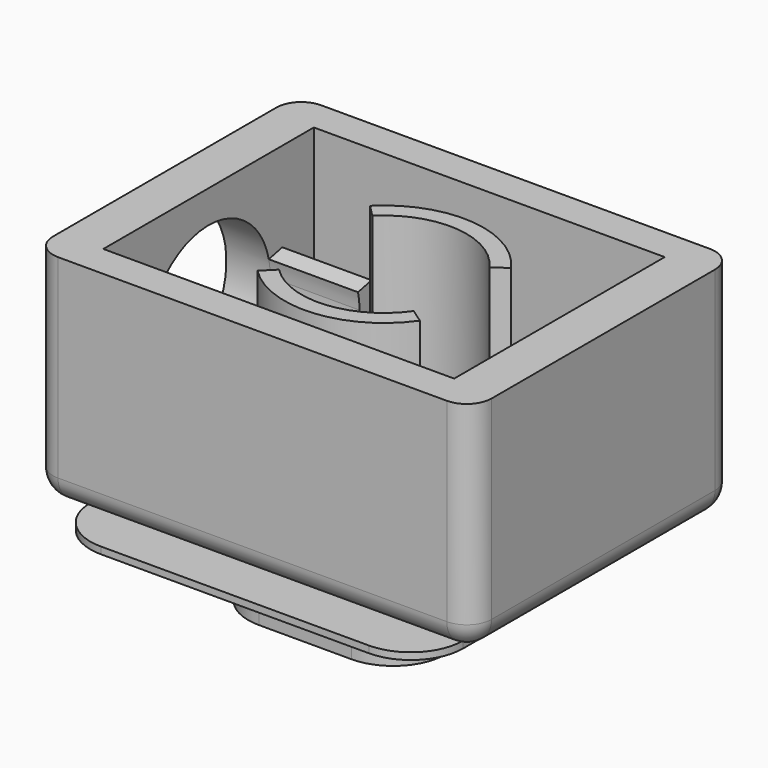
from build123d import *

# Parameters (mm, degrees)
F0_W      = 50.8
F0_H      = 38.1
F1_DEPTH  = 25.4
F2_W      = 40.64
F2_H      = 30.48
F3_DEPTH  = 22.225
F4_R      = 9.5514218063
F5_DEPTH  = 25.4
F6_R      = 8.9260934587
F7_DEPTH  = 25.4
F9_DEPTH  = 10.3378
F11_DEPTH = 21.082
F12_W     = 22.86
F12_H     = 22.86
F12_R     = 10.7189198073
F12_R_2   = 9.5514218063
F13_DEPTH = 9.6266
F14_W     = 22.86
F14_H     = 0.79375
F15_DEPTH = 10.16
F17_DEPTH = 10.16
F18_W     = 10.16
F18_H     = 0.79375
F18_W_2   = 22.86
F19_DEPTH = 10.16
F20_W     = 10.16
F20_H     = 0.79375
F20_W_2   = 22.86
F21_DEPTH = 10.16
F22_R     = 6.0707814239
F23_R     = 2.8820881508


# Not quite as in the source:
# - a length typed as a fraction of an inch, garbled in the dataset ("3 / 203.2 mm" for 3/8 in), is restored
# - a feature names something its author has since deleted; it is built from what else it names


with BuildPart() as f1:
    # F0 (on Top) → F1 (new body)
    with BuildSketch(Plane.XY):
        with Locations((-32.453101594, -1.12241521)):
            Rectangle(F0_W, F0_H)
    extrude(amount=F1_DEPTH)

    # F2 (on face) → F3 (cut)
    with BuildSketch(Plane.XY.offset(25.4)):
        with Locations((-32.453101594, -1.12241521)):
            Rectangle(F2_W, F2_H)
    extrude(amount=-F3_DEPTH, mode=Mode.SUBTRACT)

    # F4 (on face) → F5 (cut)
    with BuildSketch(Plane.XY.offset(3.175)):
        with Locations((-32.453101594, -1.12241521)):
            Circle(F4_R)
    extrude(amount=-F5_DEPTH, mode=Mode.SUBTRACT)

    # F6 (on face) → F7 (cut)
    with BuildSketch(Plane(origin=(-57.853101594, 0, 0), x_dir=(0, -1, 0), z_dir=(-1, 0, 0))):
        with Locations((1.12241521, 12.7)):
            Circle(F6_R)
    extrude(amount=-F7_DEPTH, mode=Mode.SUBTRACT)

    # F8 (on face) → F9 (join)
    with BuildSketch(Plane.YZ.offset(-52.773101594)):
        with BuildLine():
            ThreePointArc((4.2283937472, 3.175), (8.3066529455, 7.1818974988), (9.8026377187, 12.7))
            ThreePointArc((9.8026377187, 12.7), (9.7389872891, 13.8775895924), (9.5487776675, 15.0414576799))
            Line((9.5487776675, 15.0414576799), (7.5962670299, 14.6130406248))
            ThreePointArc((7.5962670299, 14.6130406248), (7.7516739529, 13.6621257514), (7.8036782487, 12.7))
            ThreePointArc((7.8036782487, 12.7), (-3.0308273005, 3.9803034613), (-9.2324659679, 16.4285682425))
            Line((-9.2324659679, 16.4285682425), (-11.0486762552, 17.2635647427))
            ThreePointArc((-11.0486762552, 17.2635647427), (-11.5132347682, 9.3254407095), (-6.4732241672, 3.175))
            Line((-6.4732241672, 3.175), (4.2283937472, 3.175))
        make_face()
    extrude(amount=F9_DEPTH)

    # F10 (on face) → F11 (join)
    with BuildSketch(Plane.XY.offset(3.175)):
        with BuildLine():
            Line((-24.6290348955, 4.3560552717), (-23.0209375751, 5.4820571376))
            ThreePointArc((-23.0209375751, 5.4820571376), (-31.4495427718, 10.3483146168), (-40.5951152599, 7.0195984558))
            Line((-40.5951152599, 7.0195984558), (-39.2069767232, 5.6314599192))
            ThreePointArc((-39.2069767232, 5.6314599192), (-31.6206403322, 8.3926605526), (-24.6290348955, 4.3560552717))
        make_face()
        with BuildLine():
            ThreePointArc((-40.5951152599, -9.2644288759), (-31.4495427718, -12.5931450369), (-23.0209375751, -7.7268875577))
            Line((-23.0209375751, -7.7268875577), (-24.6290348955, -6.6008856918))
            ThreePointArc((-24.6290348955, -6.6008856918), (-31.6206403322, -10.6374909727), (-39.2069767232, -7.8762903393))
            Line((-39.2069767232, -7.8762903393), (-40.5951152599, -9.2644288759))
        make_face()
    extrude(amount=F11_DEPTH)

    # F12 (on face) → F13 (join)
    with BuildSketch(Plane(origin=(0, 0, 0), x_dir=(1, 0, 0), z_dir=(0, 0, -1))):
        with Locations((-32.453101594, 1.12241521)):
            Rectangle(F12_W, F12_H)
        with Locations((-32.453101594, 1.12241521)):
            Circle(F12_R, mode=Mode.SUBTRACT)
        with Locations((-32.453101594, 1.12241521)):
            Circle(F12_R)
        with Locations((-32.453101594, 1.12241521)):
            Circle(F12_R_2, mode=Mode.SUBTRACT)
    extrude(amount=F13_DEPTH)

    # F14 (on face) → F15 (join)
    with BuildSketch(Plane(origin=(0, 10.30758479, 0), x_dir=(-1, 0, 0), z_dir=(0, 1, 0))):
        with Locations((32.453101594, -1.190625)):
            Rectangle(F14_W, F14_H)
    extrude(amount=F15_DEPTH)

    # F16 (on face) → F17 (join)
    with BuildSketch(Plane.YZ.offset(-21.023101594)):
        Polygon((-12.55241521, -0.79375), (-12.55241521, -1.5875), (10.30758479, -1.5875), (20.46758479, -1.5875), (20.46758479, -0.79375), (10.30758479, -0.79375), align=None)
    extrude(amount=F17_DEPTH)

    # F18 (on face) → F19 (join)
    with BuildSketch(Plane.XZ.offset(12.55241521)):
        with Locations((-15.943101594, -1.190625)):
            Rectangle(F18_W, F18_H)
        with Locations((-32.453101594, -1.190625)):
            Rectangle(F18_W_2, F18_H)
    extrude(amount=F19_DEPTH)

    # F20 (on face) → F21 (join)
    with BuildSketch(Plane(origin=(-43.883101594, 0, 0), x_dir=(0, -1, 0), z_dir=(-1, 0, 0))):
        with Locations((-15.38758479, -1.190625)):
            Rectangle(F20_W, F20_H)
        with Locations((1.12241521, -1.190625)):
            Rectangle(F20_W_2, F20_H)
        with Locations((17.63241521, -1.190625)):
            Rectangle(F20_W, F20_H)
    extrude(amount=F21_DEPTH)

    # F22
    f22_edges = [f1.edges().sort_by_distance(p)[0] for p in [
        (-10.863102, 20.467585, -1.190625),
        (-54.043102, 20.467585, -1.190625),
        (-54.043102, -22.712415, -1.190625),
        (-10.863102, -22.712415, -1.190625),
        (-21.023102, -12.552415, -5.60705),
        (-43.883102, -12.552415, -5.60705),
        (-43.883102, 10.307585, -5.60705),
        (-21.023102, 10.307585, -5.60705),
    ]]
    fillet(f22_edges, radius=F22_R)

    # F23
    f23_edges = [f1.edges().sort_by_distance(p)[0] for p in [
        (-32.453102, -20.172415, 0),
        (-57.853102, -1.122415, 0),
        (-57.853102, -20.172415, 12.7),
        (-7.053102, -1.122415, 0),
        (-7.053102, -20.172415, 12.7),
        (-32.453102, 17.927585, 0),
        (-7.053102, 17.927585, 12.7),
        (-57.853102, 17.927585, 12.7),
    ]]
    fillet(f23_edges, radius=F23_R)


solid = f1.part
